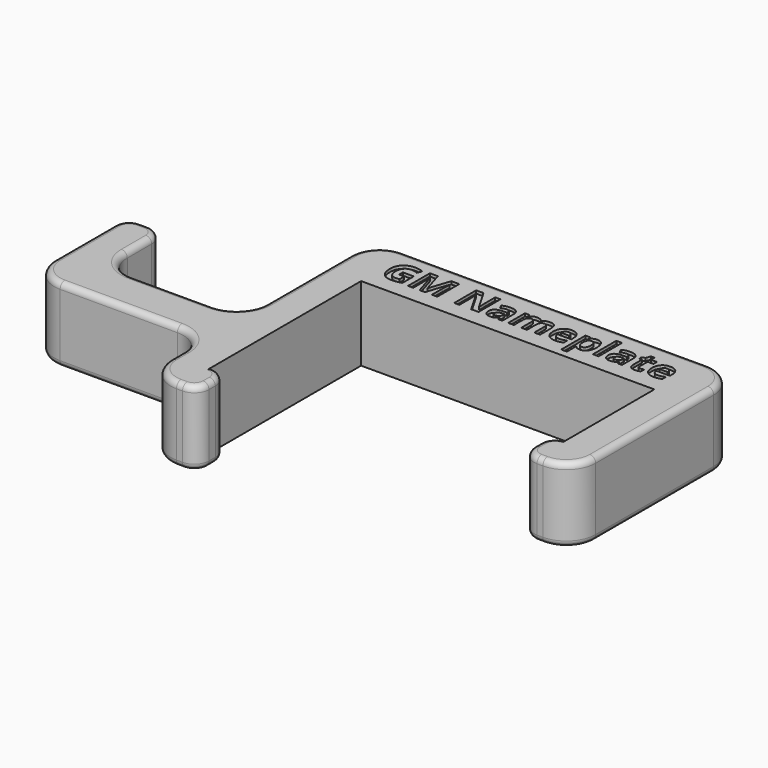
from build123d import *

# Parameters (mm, degrees)
F0_W         = 50
F0_H         = 10.16
F0_W_2       = 2.54
F0_H_2       = 6.35
F1_DEPTH     = 12.7
F2_R         = 2.5
F3_R         = 5
F4_R         = 2.53999
F5_R         = 2.54
F6_TEXT_SIZE = 6.5529068429
F7_DEPTH     = 0.5
F8_R         = 2.5
F9_T1_DEPTH  = 13.65
F9_T3_DEPTH  = 5.2
F9_T5_DEPTH  = 1.35
F9_T7_DEPTH  = 12.82
F9_T9_DEPTH  = 20
F9_T11_DEPTH = 2.7
F9_T13_DEPTH = 1.04
F9_T15_DEPTH = 1.35
F9_T17_DEPTH = 0.04
F9_T19_DEPTH = 17.94
F9_T21_DEPTH = 52
F9_T23_DEPTH = 25.16
F9_T25_DEPTH = 1
F9_T27_DEPTH = 1.27001
F9_T29_DEPTH = 1e-05
F9_T32_ANGLE = 90
F9_T34_ANGLE = 90
F9_T36_ANGLE = 90
F9_T38_ANGLE = 90
F9_T40_ANGLE = 90
F9_T42_ANGLE = 90
F9_T44_ANGLE = 90
F9_T46_ANGLE = 90
F9_T48_ANGLE = 90
F9_T50_ANGLE = 90
F9_T52_ANGLE = 90
F9_T54_ANGLE = 90
F9_T56_ANGLE = 90
F9_T58_ANGLE = 90
F9_T60_ANGLE = 90
F9_T62_ANGLE = 90
F9_T64_ANGLE = 90
F9_T66_ANGLE = 90
F9_T68_ANGLE = 90
F9_T70_ANGLE = 90
F9_T72_ANGLE = 90
F9_T74_ANGLE = 90
F9_T76_ANGLE = 90
F9_T78_ANGLE = 90
F9_T80_ANGLE = 90
F9_T82_ANGLE = 90
F9_T84_ANGLE = 90
F9_T86_ANGLE = 90


# Not quite as in the source:
# - a fillet or chamfer that OpenCascade refuses, or shapes differently, is made with other operations: its cross-section is extruded or revolved along the edge and cut away or added
# - a fillet or chamfer is up to 0.001 mm smaller than in the source, because OpenCascade refuses the exact size
# - Text() gives the source's letters only with a copy of the font that has no kerning and outlines rounded to 1/6400 em; it was checked with that copy


with BuildPart() as f1:
    # F0 (on Top) → F1 (new body)
    with BuildSketch(Plane.XY):
        with Locations((0, -5.08)):
            Rectangle(F0_W, F0_H)
        with BuildLine():
            Line((-25, -10.16), (-25, 0))
            Line((-25, 0), (-26, 0))
            ThreePointArc((-26, 0), (-29.5355339059, -1.4644660941), (-31, -5))
            Line((-31, -5), (-31, -22.94))
            ThreePointArc((-31, -22.94), (-32.4644660941, -26.4755339059), (-36, -27.94))
            Line((-36, -27.94), (-49.65, -27.94))
            ThreePointArc((-49.65, -27.94), (-53.1855339059, -26.4755339059), (-54.65, -22.94))
            Line((-54.65, -22.94), (-54.65, -15.24))
            Line((-54.65, -15.24), (-61, -15.24))
            Line((-61, -15.24), (-61, -27.94))
            Line((-61, -27.94), (-61, -30.56))
            ThreePointArc((-61, -30.56), (-59.5355339059, -34.0955339059), (-56, -35.56))
            Line((-56, -35.56), (-36, -35.56))
            ThreePointArc((-36, -35.56), (-32.4644660941, -37.0244660941), (-31, -40.56))
            Line((-31, -40.56), (-31, -43.26))
            ThreePointArc((-31, -43.26), (-29.5355339059, -46.7955339059), (-26, -48.26))
            Line((-26, -48.26), (-25, -48.26))
            Line((-25, -48.26), (-25, -41.91))
            Line((-25, -41.91), (-25, -10.16))
        make_face()
        with BuildLine():
            Line((26, 0), (25, 0))
            Line((25, 0), (25, -10.16))
            Line((25, -10.16), (25, -28.81))
            Line((25, -28.81), (25, -35.16))
            Line((25, -35.16), (31, -35.16))
            Line((31, -35.16), (31, -5))
            ThreePointArc((31, -5), (29.5355339059, -1.4644660941), (26, 0))
        make_face()
        with Locations((-23.73, -45.085)):
            Rectangle(F0_W_2, F0_H_2)
        with Locations((23.73, -31.985)):
            Rectangle(F0_W_2, F0_H_2)
    extrude(amount=F1_DEPTH)

    # F2
    f2_edges = [f1.edges().sort_by_distance(p)[0] for p in [
        (-61, -15.24, 6.35),
        (-54.65, -15.24, 6.35),
    ]]
    fillet(f2_edges, radius=F2_R)

    # F3
    f3_edges = [f1.edges().sort_by_distance(p)[0] for p in [
        (31, -35.16, 6.35),
    ]]
    fillet(f3_edges, radius=F3_R)

    # F4 (radius 2.54 in the source; OpenCascade refuses exactly that, so slightly less here)
    f4_edges = [f1.edges().sort_by_distance(p)[0] for p in [
        (22.46, -28.81, 6.35),
    ]]
    fillet(f4_edges, radius=F4_R)

    # F5
    f5_edges = [f1.edges().sort_by_distance(p)[0] for p in [
        (22.46, -35.16, 6.35),
    ]]
    fillet(f5_edges, radius=F5_R)

    # F6 (on face) → F7 (cut)
    with BuildSketch(Plane.XY.offset(12.7)):
        with Locations((-24.5902948737, -7.3492400115)):
            Text('GM Nameplate', F6_TEXT_SIZE, font='Open Sans', font_style=FontStyle.BOLD, text_align=(TextAlign.LEFT, TextAlign.BOTTOM))
    extrude(amount=-F7_DEPTH, mode=Mode.SUBTRACT)

    # F8
    f8_edges = [f1.edges().sort_by_distance(p)[0] for p in [
        (-22.46, -41.91, 6.35),
        (-22.46, -48.26, 6.35),
    ]]
    fillet(f8_edges, radius=F8_R)

    # F9: fillet of radius 1 on 12 edges, made by hand

    # F9_s2 → F9_t1 (cut)
    with BuildSketch(Plane.YZ.offset(-49.65)):
        with BuildLine():
            ThreePointArc((-28.94, 0), (-28.2328932188, 0.2928932188), (-27.94, 1))
            Line((-27.94, 1), (-27.94, 0))
            Line((-27.94, 0), (-28.94, 0))
        make_face()
        with BuildLine():
            ThreePointArc((-27.94, 11.7), (-28.2328932188, 12.4071067812), (-28.94, 12.7))
            Line((-28.94, 12.7), (-27.94, 12.7))
            Line((-27.94, 12.7), (-27.94, 11.7))
        make_face()
    extrude(amount=F9_T1_DEPTH, mode=Mode.SUBTRACT)

    # F9_s4 → F9_t3 (cut)
    with BuildSketch(Plane.XZ.offset(17.74)):
        with BuildLine():
            ThreePointArc((-55.65, 0), (-54.9428932188, 0.2928932188), (-54.65, 1))
            Line((-54.65, 1), (-54.65, 0))
            Line((-54.65, 0), (-55.65, 0))
        make_face()
        with BuildLine():
            ThreePointArc((-54.65, 11.7), (-54.9428932188, 12.4071067812), (-55.65, 12.7))
            Line((-55.65, 12.7), (-54.65, 12.7))
            Line((-54.65, 12.7), (-54.65, 11.7))
        make_face()
    extrude(amount=F9_T3_DEPTH, mode=Mode.SUBTRACT)

    # F9_s6 → F9_t5 (cut)
    with BuildSketch(Plane.YZ.offset(-58.5)):
        with BuildLine():
            ThreePointArc((-16.24, 0), (-15.5328932188, 0.2928932188), (-15.24, 1))
            Line((-15.24, 1), (-15.24, 0))
            Line((-15.24, 0), (-16.24, 0))
        make_face()
        with BuildLine():
            ThreePointArc((-15.24, 11.7), (-15.5328932188, 12.4071067812), (-16.24, 12.7))
            Line((-16.24, 12.7), (-15.24, 12.7))
            Line((-15.24, 12.7), (-15.24, 11.7))
        make_face()
    extrude(amount=F9_T5_DEPTH, mode=Mode.SUBTRACT)

    # F9_s8 → F9_t7 (cut)
    with BuildSketch(Plane.XZ.offset(17.74)):
        with BuildLine():
            ThreePointArc((-61, 11.7), (-60.7071067812, 12.4071067812), (-60, 12.7))
            Line((-60, 12.7), (-61, 12.7))
            Line((-61, 12.7), (-61, 11.7))
        make_face()
        with BuildLine():
            ThreePointArc((-60, 0), (-60.7071067812, 0.2928932188), (-61, 1))
            Line((-61, 1), (-61, 0))
            Line((-61, 0), (-60, 0))
        make_face()
    extrude(amount=F9_T7_DEPTH, mode=Mode.SUBTRACT)

    # F9_s10 → F9_t9 (cut)
    with BuildSketch(Plane.YZ.offset(-56)):
        with BuildLine():
            ThreePointArc((-35.56, 11.7), (-35.2671067812, 12.4071067812), (-34.56, 12.7))
            Line((-34.56, 12.7), (-35.56, 12.7))
            Line((-35.56, 12.7), (-35.56, 11.7))
        make_face()
        with BuildLine():
            ThreePointArc((-34.56, 0), (-35.2671067812, 0.2928932188), (-35.56, 1))
            Line((-35.56, 1), (-35.56, 0))
            Line((-35.56, 0), (-34.56, 0))
        make_face()
    extrude(amount=F9_T9_DEPTH, mode=Mode.SUBTRACT)

    # F9_s12 → F9_t11 (cut)
    with BuildSketch(Plane.XZ.offset(40.56)):
        with BuildLine():
            ThreePointArc((-31, 11.7), (-30.7071067812, 12.4071067812), (-30, 12.7))
            Line((-30, 12.7), (-31, 12.7))
            Line((-31, 12.7), (-31, 11.7))
        make_face()
        with BuildLine():
            ThreePointArc((-30, 0), (-30.7071067812, 0.2928932188), (-31, 1))
            Line((-31, 1), (-31, 0))
            Line((-31, 0), (-30, 0))
        make_face()
    extrude(amount=F9_T11_DEPTH, mode=Mode.SUBTRACT)

    # F9_s14 → F9_t13 (cut)
    with BuildSketch(Plane.YZ.offset(-26)):
        with BuildLine():
            ThreePointArc((-48.26, 11.7), (-47.9671067812, 12.4071067812), (-47.26, 12.7))
            Line((-47.26, 12.7), (-48.26, 12.7))
            Line((-48.26, 12.7), (-48.26, 11.7))
        make_face()
        with BuildLine():
            ThreePointArc((-47.26, 0), (-47.9671067812, 0.2928932188), (-48.26, 1))
            Line((-48.26, 1), (-48.26, 0))
            Line((-48.26, 0), (-47.26, 0))
        make_face()
    extrude(amount=F9_T13_DEPTH, mode=Mode.SUBTRACT)

    # F9_s16 → F9_t15 (cut)
    with BuildSketch(Plane.XZ.offset(44.41)):
        with BuildLine():
            ThreePointArc((-22.46, 11.7), (-22.7528932188, 12.4071067812), (-23.46, 12.7))
            Line((-23.46, 12.7), (-22.46, 12.7))
            Line((-22.46, 12.7), (-22.46, 11.7))
        make_face()
        with BuildLine():
            ThreePointArc((-23.46, 0), (-22.7528932188, 0.2928932188), (-22.46, 1))
            Line((-22.46, 1), (-22.46, 0))
            Line((-22.46, 0), (-23.46, 0))
        make_face()
    extrude(amount=F9_T15_DEPTH, mode=Mode.SUBTRACT)

    # F9_s18 → F9_t17 (cut)
    with BuildSketch(Plane.YZ.offset(-25)):
        with BuildLine():
            ThreePointArc((-41.91, 11.7), (-42.2028932188, 12.4071067812), (-42.91, 12.7))
            Line((-42.91, 12.7), (-41.91, 12.7))
            Line((-41.91, 12.7), (-41.91, 11.7))
        make_face()
        with BuildLine():
            ThreePointArc((-42.91, 0), (-42.2028932188, 0.2928932188), (-41.91, 1))
            Line((-41.91, 1), (-41.91, 0))
            Line((-41.91, 0), (-42.91, 0))
        make_face()
    extrude(amount=F9_T17_DEPTH, mode=Mode.SUBTRACT)

    # F9_s20 → F9_t19 (cut)
    with BuildSketch(Plane.XZ.offset(5)):
        with BuildLine():
            ThreePointArc((-31, 11.7), (-30.7071067812, 12.4071067812), (-30, 12.7))
            Line((-30, 12.7), (-31, 12.7))
            Line((-31, 12.7), (-31, 11.7))
        make_face()
        with BuildLine():
            ThreePointArc((-30, 0), (-30.7071067812, 0.2928932188), (-31, 1))
            Line((-31, 1), (-31, 0))
            Line((-31, 0), (-30, 0))
        make_face()
    extrude(amount=F9_T19_DEPTH, mode=Mode.SUBTRACT)

    # F9_s22 → F9_t21 (cut)
    with BuildSketch(Plane.YZ.offset(-26)):
        with BuildLine():
            ThreePointArc((0, 11.7), (-0.2928932188, 12.4071067812), (-1, 12.7))
            Line((-1, 12.7), (0, 12.7))
            Line((0, 12.7), (0, 11.7))
        make_face()
        with BuildLine():
            ThreePointArc((-1, 0), (-0.2928932188, 0.2928932188), (0, 1))
            Line((0, 1), (0, 0))
            Line((0, 0), (-1, 0))
        make_face()
    extrude(amount=F9_T21_DEPTH, mode=Mode.SUBTRACT)

    # F9_s24 → F9_t23 (cut)
    with BuildSketch(Plane.XZ.offset(5)):
        with BuildLine():
            ThreePointArc((31, 11.7), (30.7071067812, 12.4071067812), (30, 12.7))
            Line((30, 12.7), (31, 12.7))
            Line((31, 12.7), (31, 11.7))
        make_face()
        with BuildLine():
            ThreePointArc((30, 0), (30.7071067812, 0.2928932188), (31, 1))
            Line((31, 1), (31, 0))
            Line((31, 0), (30, 0))
        make_face()
    extrude(amount=F9_T23_DEPTH, mode=Mode.SUBTRACT)

    # F9_s26 → F9_t25 (cut)
    with BuildSketch(Plane.YZ.offset(25)):
        with BuildLine():
            ThreePointArc((-35.16, 11.7), (-34.8671067812, 12.4071067812), (-34.16, 12.7))
            Line((-34.16, 12.7), (-35.16, 12.7))
            Line((-35.16, 12.7), (-35.16, 11.7))
        make_face()
        with BuildLine():
            ThreePointArc((-34.16, 0), (-34.8671067812, 0.2928932188), (-35.16, 1))
            Line((-35.16, 1), (-35.16, 0))
            Line((-35.16, 0), (-34.16, 0))
        make_face()
    extrude(amount=F9_T25_DEPTH, mode=Mode.SUBTRACT)

    # F9_s28 → F9_t27 (cut)
    with BuildSketch(Plane.XZ.offset(31.34999)):
        with BuildLine():
            ThreePointArc((22.46, 11.7), (22.7528932188, 12.4071067812), (23.46, 12.7))
            Line((23.46, 12.7), (22.46, 12.7))
            Line((22.46, 12.7), (22.46, 11.7))
        make_face()
        with BuildLine():
            ThreePointArc((23.46, 0), (22.7528932188, 0.2928932188), (22.46, 1))
            Line((22.46, 1), (22.46, 0))
            Line((22.46, 0), (23.46, 0))
        make_face()
    extrude(amount=F9_T27_DEPTH, mode=Mode.SUBTRACT)

    # F9_s30 → F9_t29 (cut)
    with BuildSketch(Plane.YZ.offset(24.99999)):
        with BuildLine():
            ThreePointArc((-28.81, 11.7), (-29.1028932188, 12.4071067812), (-29.81, 12.7))
            Line((-29.81, 12.7), (-28.81, 12.7))
            Line((-28.81, 12.7), (-28.81, 11.7))
        make_face()
        with BuildLine():
            ThreePointArc((-29.81, 0), (-29.1028932188, 0.2928932188), (-28.81, 1))
            Line((-28.81, 1), (-28.81, 0))
            Line((-28.81, 0), (-29.81, 0))
        make_face()
    extrude(amount=F9_T29_DEPTH, mode=Mode.SUBTRACT)

    # F9_s31 → F9_t32 (revolve, cut)
    with BuildSketch(Plane.YZ.offset(-49.65)):
        with BuildLine():
            ThreePointArc((-28.94, 0), (-28.2328932188, 0.2928932188), (-27.94, 1))
            Line((-27.94, 1), (-27.94, 0))
            Line((-27.94, 0), (-28.94, 0))
        make_face()
    revolve(axis=Axis((-49.65, -22.94, 0), (0, 0, -1)), revolution_arc=F9_T32_ANGLE, mode=Mode.SUBTRACT)

    # F9_s33 → F9_t34 (revolve, cut)
    with BuildSketch(Plane.YZ.offset(-49.65)):
        with BuildLine():
            ThreePointArc((-27.94, 11.7), (-28.2328932188, 12.4071067812), (-28.94, 12.7))
            Line((-28.94, 12.7), (-27.94, 12.7))
            Line((-27.94, 12.7), (-27.94, 11.7))
        make_face()
    revolve(axis=Axis((-49.65, -22.94, 12.7), (0, 0, -1)), revolution_arc=F9_T34_ANGLE, mode=Mode.SUBTRACT)

    # F9_s35 → F9_t36 (revolve, cut)
    with BuildSketch(Plane.XZ.offset(17.74)):
        with BuildLine():
            ThreePointArc((-55.65, 0), (-54.9428932188, 0.2928932188), (-54.65, 1))
            Line((-54.65, 1), (-54.65, 0))
            Line((-54.65, 0), (-55.65, 0))
        make_face()
    revolve(axis=Axis((-57.15, -17.74, 0), (0, 0, 1)), revolution_arc=F9_T36_ANGLE, mode=Mode.SUBTRACT)

    # F9_s37 → F9_t38 (revolve, cut)
    with BuildSketch(Plane.YZ.offset(-58.5)):
        with BuildLine():
            ThreePointArc((-16.24, 0), (-15.5328932188, 0.2928932188), (-15.24, 1))
            Line((-15.24, 1), (-15.24, 0))
            Line((-15.24, 0), (-16.24, 0))
        make_face()
    revolve(axis=Axis((-58.5, -17.74, 0), (0, 0, 1)), revolution_arc=F9_T38_ANGLE, mode=Mode.SUBTRACT)

    # F9_s39 → F9_t40 (revolve, cut)
    with BuildSketch(Plane.YZ.offset(-58.5)):
        with BuildLine():
            ThreePointArc((-15.24, 11.7), (-15.5328932188, 12.4071067812), (-16.24, 12.7))
            Line((-16.24, 12.7), (-15.24, 12.7))
            Line((-15.24, 12.7), (-15.24, 11.7))
        make_face()
    revolve(axis=Axis((-58.5, -17.74, 12.7), (0, 0, 1)), revolution_arc=F9_T40_ANGLE, mode=Mode.SUBTRACT)

    # F9_s41 → F9_t42 (revolve, cut)
    with BuildSketch(Plane.XZ.offset(17.74)):
        with BuildLine():
            ThreePointArc((-54.65, 11.7), (-54.9428932188, 12.4071067812), (-55.65, 12.7))
            Line((-55.65, 12.7), (-54.65, 12.7))
            Line((-54.65, 12.7), (-54.65, 11.7))
        make_face()
    revolve(axis=Axis((-57.15, -17.74, 12.7), (0, 0, 1)), revolution_arc=F9_T42_ANGLE, mode=Mode.SUBTRACT)

    # F9_s43 → F9_t44 (revolve, cut)
    with BuildSketch(Plane.XZ.offset(30.56)):
        with BuildLine():
            ThreePointArc((-61, 11.7), (-60.7071067812, 12.4071067812), (-60, 12.7))
            Line((-60, 12.7), (-61, 12.7))
            Line((-61, 12.7), (-61, 11.7))
        make_face()
    revolve(axis=Axis((-56, -30.56, 12.7), (0, 0, 1)), revolution_arc=F9_T44_ANGLE, mode=Mode.SUBTRACT)

    # F9_s45 → F9_t46 (revolve, cut)
    with BuildSketch(Plane.YZ.offset(-36)):
        with BuildLine():
            ThreePointArc((-35.56, 11.7), (-35.2671067812, 12.4071067812), (-34.56, 12.7))
            Line((-34.56, 12.7), (-35.56, 12.7))
            Line((-35.56, 12.7), (-35.56, 11.7))
        make_face()
    revolve(axis=Axis((-36, -40.56, 12.7), (0, 0, -1)), revolution_arc=F9_T46_ANGLE, mode=Mode.SUBTRACT)

    # F9_s47 → F9_t48 (revolve, cut)
    with BuildSketch(Plane.XZ.offset(43.26)):
        with BuildLine():
            ThreePointArc((-31, 11.7), (-30.7071067812, 12.4071067812), (-30, 12.7))
            Line((-30, 12.7), (-31, 12.7))
            Line((-31, 12.7), (-31, 11.7))
        make_face()
    revolve(axis=Axis((-26, -43.26, 12.7), (0, 0, 1)), revolution_arc=F9_T48_ANGLE, mode=Mode.SUBTRACT)

    # F9_s49 → F9_t50 (revolve, cut)
    with BuildSketch(Plane.XZ.offset(45.76)):
        with BuildLine():
            ThreePointArc((-22.46, 11.7), (-22.7528932188, 12.4071067812), (-23.46, 12.7))
            Line((-23.46, 12.7), (-22.46, 12.7))
            Line((-22.46, 12.7), (-22.46, 11.7))
        make_face()
    revolve(axis=Axis((-24.96, -45.76, 12.7), (0, 0, -1)), revolution_arc=F9_T50_ANGLE, mode=Mode.SUBTRACT)

    # F9_s51 → F9_t52 (revolve, cut)
    with BuildSketch(Plane.YZ.offset(-24.96)):
        with BuildLine():
            ThreePointArc((-41.91, 11.7), (-42.2028932188, 12.4071067812), (-42.91, 12.7))
            Line((-42.91, 12.7), (-41.91, 12.7))
            Line((-41.91, 12.7), (-41.91, 11.7))
        make_face()
    revolve(axis=Axis((-24.96, -44.41, 12.7), (0, 0, -1)), revolution_arc=F9_T52_ANGLE, mode=Mode.SUBTRACT)

    # F9_s53 → F9_t54 (revolve, cut)
    with BuildSketch(Plane.XZ.offset(30.56)):
        with BuildLine():
            ThreePointArc((-60, 0), (-60.7071067812, 0.2928932188), (-61, 1))
            Line((-61, 1), (-61, 0))
            Line((-61, 0), (-60, 0))
        make_face()
    revolve(axis=Axis((-56, -30.56, 0), (0, 0, 1)), revolution_arc=F9_T54_ANGLE, mode=Mode.SUBTRACT)

    # F9_s55 → F9_t56 (revolve, cut)
    with BuildSketch(Plane.YZ.offset(-36)):
        with BuildLine():
            ThreePointArc((-34.56, 0), (-35.2671067812, 0.2928932188), (-35.56, 1))
            Line((-35.56, 1), (-35.56, 0))
            Line((-35.56, 0), (-34.56, 0))
        make_face()
    revolve(axis=Axis((-36, -40.56, 0), (0, 0, -1)), revolution_arc=F9_T56_ANGLE, mode=Mode.SUBTRACT)

    # F9_s57 → F9_t58 (revolve, cut)
    with BuildSketch(Plane.XZ.offset(43.26)):
        with BuildLine():
            ThreePointArc((-30, 0), (-30.7071067812, 0.2928932188), (-31, 1))
            Line((-31, 1), (-31, 0))
            Line((-31, 0), (-30, 0))
        make_face()
    revolve(axis=Axis((-26, -43.26, 0), (0, 0, 1)), revolution_arc=F9_T58_ANGLE, mode=Mode.SUBTRACT)

    # F9_s59 → F9_t60 (revolve, cut)
    with BuildSketch(Plane.XZ.offset(45.76)):
        with BuildLine():
            ThreePointArc((-23.46, 0), (-22.7528932188, 0.2928932188), (-22.46, 1))
            Line((-22.46, 1), (-22.46, 0))
            Line((-22.46, 0), (-23.46, 0))
        make_face()
    revolve(axis=Axis((-24.96, -45.76, 0), (0, 0, -1)), revolution_arc=F9_T60_ANGLE, mode=Mode.SUBTRACT)

    # F9_s61 → F9_t62 (revolve, cut)
    with BuildSketch(Plane.YZ.offset(-24.96)):
        with BuildLine():
            ThreePointArc((-42.91, 0), (-42.2028932188, 0.2928932188), (-41.91, 1))
            Line((-41.91, 1), (-41.91, 0))
            Line((-41.91, 0), (-42.91, 0))
        make_face()
    revolve(axis=Axis((-24.96, -44.41, 0), (0, 0, -1)), revolution_arc=F9_T62_ANGLE, mode=Mode.SUBTRACT)

    # F9_s63 → F9_t64 (revolve, cut)
    with BuildSketch(Plane.XZ.offset(22.94)):
        with BuildLine():
            ThreePointArc((-31, 11.7), (-30.7071067812, 12.4071067812), (-30, 12.7))
            Line((-30, 12.7), (-31, 12.7))
            Line((-31, 12.7), (-31, 11.7))
        make_face()
    revolve(axis=Axis((-36, -22.94, 12.7), (0, 0, -1)), revolution_arc=F9_T64_ANGLE, mode=Mode.SUBTRACT)

    # F9_s65 → F9_t66 (revolve, cut)
    with BuildSketch(Plane.YZ.offset(-26)):
        with BuildLine():
            ThreePointArc((0, 11.7), (-0.2928932188, 12.4071067812), (-1, 12.7))
            Line((-1, 12.7), (0, 12.7))
            Line((0, 12.7), (0, 11.7))
        make_face()
    revolve(axis=Axis((-26, -5, 12.7), (0, 0, 1)), revolution_arc=F9_T66_ANGLE, mode=Mode.SUBTRACT)

    # F9_s67 → F9_t68 (revolve, cut)
    with BuildSketch(Plane.XZ.offset(5)):
        with BuildLine():
            ThreePointArc((31, 11.7), (30.7071067812, 12.4071067812), (30, 12.7))
            Line((30, 12.7), (31, 12.7))
            Line((31, 12.7), (31, 11.7))
        make_face()
    revolve(axis=Axis((26, -5, 12.7), (0, 0, 1)), revolution_arc=F9_T68_ANGLE, mode=Mode.SUBTRACT)

    # F9_s69 → F9_t70 (revolve, cut)
    with BuildSketch(Plane.XZ.offset(30.16)):
        with BuildLine():
            ThreePointArc((31, 11.7), (30.7071067812, 12.4071067812), (30, 12.7))
            Line((30, 12.7), (31, 12.7))
            Line((31, 12.7), (31, 11.7))
        make_face()
    revolve(axis=Axis((26, -30.16, 12.7), (0, 0, -1)), revolution_arc=F9_T70_ANGLE, mode=Mode.SUBTRACT)

    # F9_s71 → F9_t72 (revolve, cut)
    with BuildSketch(Plane.XZ.offset(32.62)):
        with BuildLine():
            ThreePointArc((22.46, 11.7), (22.7528932188, 12.4071067812), (23.46, 12.7))
            Line((23.46, 12.7), (22.46, 12.7))
            Line((22.46, 12.7), (22.46, 11.7))
        make_face()
    revolve(axis=Axis((25, -32.62, 12.7), (0, 0, 1)), revolution_arc=F9_T72_ANGLE, mode=Mode.SUBTRACT)

    # F9_s73 → F9_t74 (revolve, cut)
    with BuildSketch(Plane.XZ.offset(31.34999)):
        with BuildLine():
            ThreePointArc((22.46, 11.7), (22.7528932188, 12.4071067812), (23.46, 12.7))
            Line((23.46, 12.7), (22.46, 12.7))
            Line((22.46, 12.7), (22.46, 11.7))
        make_face()
    revolve(axis=Axis((24.99999, -31.34999, 12.7), (0, 0, -1)), revolution_arc=F9_T74_ANGLE, mode=Mode.SUBTRACT)

    # F9_s75 → F9_t76 (revolve, cut)
    with BuildSketch(Plane.XZ.offset(22.94)):
        with BuildLine():
            ThreePointArc((-30, 0), (-30.7071067812, 0.2928932188), (-31, 1))
            Line((-31, 1), (-31, 0))
            Line((-31, 0), (-30, 0))
        make_face()
    revolve(axis=Axis((-36, -22.94, 0), (0, 0, -1)), revolution_arc=F9_T76_ANGLE, mode=Mode.SUBTRACT)

    # F9_s77 → F9_t78 (revolve, cut)
    with BuildSketch(Plane.YZ.offset(-26)):
        with BuildLine():
            ThreePointArc((-1, 0), (-0.2928932188, 0.2928932188), (0, 1))
            Line((0, 1), (0, 0))
            Line((0, 0), (-1, 0))
        make_face()
    revolve(axis=Axis((-26, -5, 0), (0, 0, 1)), revolution_arc=F9_T78_ANGLE, mode=Mode.SUBTRACT)

    # F9_s79 → F9_t80 (revolve, cut)
    with BuildSketch(Plane.XZ.offset(5)):
        with BuildLine():
            ThreePointArc((30, 0), (30.7071067812, 0.2928932188), (31, 1))
            Line((31, 1), (31, 0))
            Line((31, 0), (30, 0))
        make_face()
    revolve(axis=Axis((26, -5, 0), (0, 0, 1)), revolution_arc=F9_T80_ANGLE, mode=Mode.SUBTRACT)

    # F9_s81 → F9_t82 (revolve, cut)
    with BuildSketch(Plane.XZ.offset(30.16)):
        with BuildLine():
            ThreePointArc((30, 0), (30.7071067812, 0.2928932188), (31, 1))
            Line((31, 1), (31, 0))
            Line((31, 0), (30, 0))
        make_face()
    revolve(axis=Axis((26, -30.16, 0), (0, 0, -1)), revolution_arc=F9_T82_ANGLE, mode=Mode.SUBTRACT)

    # F9_s83 → F9_t84 (revolve, cut)
    with BuildSketch(Plane.XZ.offset(32.62)):
        with BuildLine():
            ThreePointArc((23.46, 0), (22.7528932188, 0.2928932188), (22.46, 1))
            Line((22.46, 1), (22.46, 0))
            Line((22.46, 0), (23.46, 0))
        make_face()
    revolve(axis=Axis((25, -32.62, 0), (0, 0, 1)), revolution_arc=F9_T84_ANGLE, mode=Mode.SUBTRACT)

    # F9_s85 → F9_t86 (revolve, cut)
    with BuildSketch(Plane.XZ.offset(31.34999)):
        with BuildLine():
            ThreePointArc((23.46, 0), (22.7528932188, 0.2928932188), (22.46, 1))
            Line((22.46, 1), (22.46, 0))
            Line((22.46, 0), (23.46, 0))
        make_face()
    revolve(axis=Axis((24.99999, -31.34999, 0), (0, 0, -1)), revolution_arc=F9_T86_ANGLE, mode=Mode.SUBTRACT)


solid = f1.part
